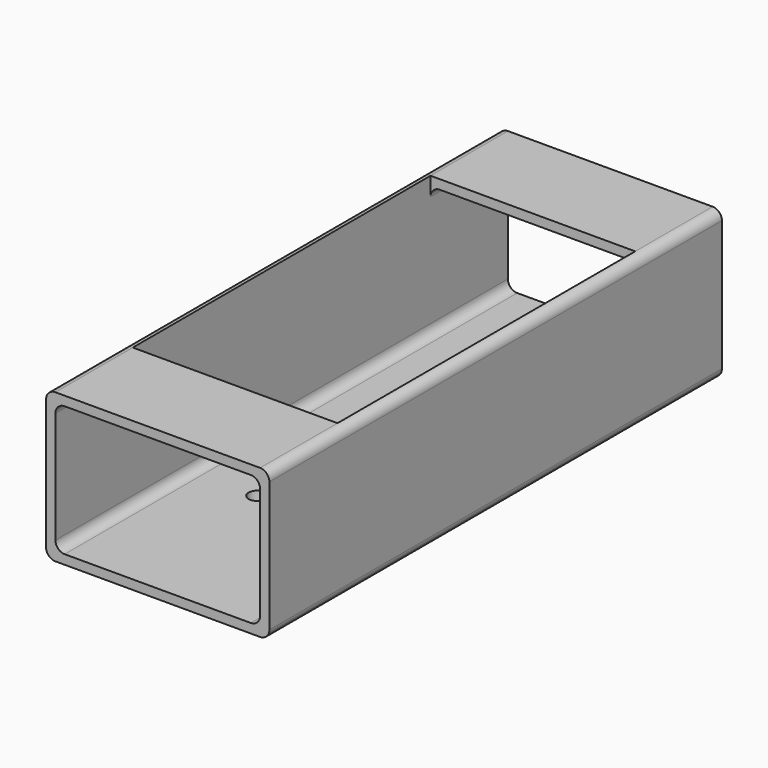
from build123d import *

# Parameters (mm, degrees)
F0_W     = 76.2
F0_H     = 50.8
F0_W_2   = 69.85
F0_H_2   = 44.45
F2_DEPTH = 193.04
F3_R     = 3.175
F4_R     = 3
F5_DEPTH = 25.4
F7_DEPTH = 25.4


# Not quite as in the source:
# - a variable given as a bare number and used for a length is read in inches; the dataset says mm whatever the document's units were


with BuildPart() as f2:
    # F0 (on Front) → F2 (new body)
    with BuildSketch(Plane.XZ):
        Rectangle(F0_W, F0_H)
        Rectangle(F0_W_2, F0_H_2, mode=Mode.SUBTRACT)
    extrude(amount=F2_DEPTH)

    # F3
    f3_edges = [f2.edges().sort_by_distance(p)[0] for p in [
        (-38.1, -96.52, -25.4),
        (-38.1, -96.52, 25.4),
        (38.1, -96.52, -25.4),
        (38.1, -96.52, 25.4),
        (-34.925, -96.52, -22.225),
        (-34.925, -96.52, 22.225),
        (34.925, -96.52, 22.225),
        (34.925, -96.52, -22.225),
    ]]
    fillet(f3_edges, radius=F3_R)

    # F4 (on face) → F5 (cut)
    with BuildSketch(Plane(origin=(0, 0, -25.4), x_dir=(1, 0, 0), z_dir=(0, 0, -1))):
        with Locations((-12.7, 58.42)):
            Circle(F4_R)
        with Locations((12.7, 58.42)):
            Circle(F4_R)
        with Locations((12.7, 134.62)):
            Circle(F4_R)
        with Locations((-12.7, 134.62)):
            Circle(F4_R)
    extrude(amount=-F5_DEPTH, mode=Mode.SUBTRACT)

    # F6 (on face) → F7 (cut)
    with BuildSketch(Plane.XY.offset(25.4)):
        Polygon((34.925, -33.02), (0, -33.02), (-34.925, -33.02), (-34.925, -160.02), (34.925, -160.02), align=None)
    extrude(amount=-F7_DEPTH, mode=Mode.SUBTRACT)


solid = f2.part
